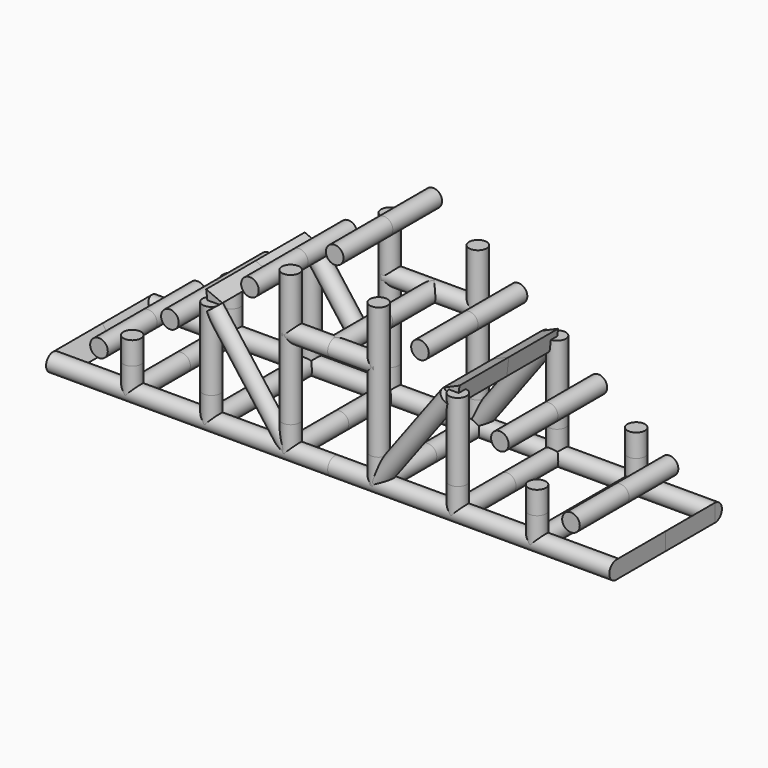
from build123d import *

# Parameters (mm, degrees)
F0_R      = 1.27
F1_DEPTH  = 40.64
F2_DEPTH  = 40.64
F3_R      = 1.27
F4_DEPTH  = 3.81
F6_DEPTH  = 8.89
F7_DEPTH  = 8.89
F11_DEPTH = 8.89
F12_DEPTH = 8.89
F16_DEPTH = 3.302
F17_DEPTH = 11.2522
F18_DEPTH = 19.0246
F5_R      = 1.27
F19_DEPTH = 8.89
F20_DEPTH = 8.89
F21_R     = 1.27
F22_DEPTH = 8.89
F23_DEPTH = 8.89
F24_R     = 1.27
F25_DEPTH = 6.604
F26_DEPTH = 6.604
F27_DEPTH = 8.89
F28_DEPTH = 8.89
F29_R     = 1.2711248992
F30_DEPTH = 17.78
F32_DEPTH = 17.78
F31_R     = 1.27
F33_R     = 1.27
F34_DEPTH = 8.89
F35_DEPTH = 8.89


# Not quite as in the source:
# - the program builds the solid bodies; features that only make, move or delete a surface that nothing else refers to are left out


with BuildPart() as f1:
    # F0 (on Right) → F1 (new body)
    with BuildSketch(Plane.YZ):
        with Locations((-8.89, 0)):
            Circle(F0_R)
    extrude(amount=F1_DEPTH)

    # F5 (on Front) → F11 (join)
    with BuildSketch(Plane.XZ):
        Polygon((40.64, -1.2507883366), (40.64, 1.2892116634), (38.9128, -1.2507883366), align=None)
    extrude(amount=F11_DEPTH)


with BuildPart() as f1b:
    # F0 (on Right) → F1, piece 2 (new body)
    with BuildSketch(Plane.YZ):
        with Locations((8.89, 0)):
            Circle(F0_R)
    extrude(amount=F1_DEPTH)


with BuildPart() as f2:
    # F0 (on Right) → F2 (new body)
    with BuildSketch(Plane.YZ):
        with Locations((-8.89, 0)):
            Circle(F0_R)
    extrude(amount=-F2_DEPTH)

    # F5 (on Front) → F6 (join)
    with BuildSketch(Plane.XZ):
        Polygon((-38.9128, -1.2715099968), (-40.64, 1.2684900032), (-40.64, -1.2715099968), align=None)
    extrude(amount=F6_DEPTH)


with BuildPart() as f2b:
    # F0 (on Right) → F2, piece 2 (new body)
    with BuildSketch(Plane.YZ):
        with Locations((8.89, 0)):
            Circle(F0_R)
    extrude(amount=-F2_DEPTH)


with BuildPart() as f4:
    # F3 (on Top) → F4 (new body)
    with BuildSketch(Plane.XY):
        with Locations((-29.21, -8.8966675103)):
            Circle(F3_R)
    extrude(amount=F4_DEPTH)


with BuildPart() as f4b:
    # F3 (on Top) → F4, piece 2 (new body)
    with BuildSketch(Plane.XY):
        with Locations((-17.78, -8.8966675103)):
            Circle(F3_R)
    extrude(amount=F4_DEPTH)


with BuildPart() as f4c:
    # F3 (on Top) → F4, piece 3 (new body)
    with BuildSketch(Plane.XY):
        with Locations((-6.35, -8.8966675103)):
            Circle(F3_R)
    extrude(amount=F4_DEPTH)


with BuildPart() as f4d:
    # F3 (on Top) → F4, piece 4 (new body)
    with BuildSketch(Plane.XY):
        with Locations((6.35, -8.8966675103)):
            Circle(F3_R)
    extrude(amount=F4_DEPTH)


with BuildPart() as f4e:
    # F3 (on Top) → F4, piece 5 (new body)
    with BuildSketch(Plane.XY):
        with Locations((17.78, -8.8966675103)):
            Circle(F3_R)
    extrude(amount=F4_DEPTH)


with BuildPart() as f4f:
    # F3 (on Top) → F4, piece 6 (new body)
    with BuildSketch(Plane.XY):
        with Locations((29.21, -8.8966675103)):
            Circle(F3_R)
    extrude(amount=F4_DEPTH)


with BuildPart() as f4g:
    # F3 (on Top) → F4, piece 7 (new body)
    with BuildSketch(Plane.XY):
        with Locations((29.21, 8.99035763)):
            Circle(F3_R)
    extrude(amount=F4_DEPTH)


with BuildPart() as f4h:
    # F3 (on Top) → F4, piece 8 (new body)
    with BuildSketch(Plane.XY):
        with Locations((17.78, 8.99035763)):
            Circle(F3_R)
    extrude(amount=F4_DEPTH)


with BuildPart() as f4i:
    # F3 (on Top) → F4, piece 9 (new body)
    with BuildSketch(Plane.XY):
        with Locations((6.35, 8.99035763)):
            Circle(F3_R)
    extrude(amount=F4_DEPTH)


with BuildPart() as f4j:
    # F3 (on Top) → F4, piece 10 (new body)
    with BuildSketch(Plane.XY):
        with Locations((-6.35, 8.99035763)):
            Circle(F3_R)
    extrude(amount=F4_DEPTH)


with BuildPart() as f4k:
    # F3 (on Top) → F4, piece 11 (new body)
    with BuildSketch(Plane.XY):
        with Locations((-17.78, 8.99035763)):
            Circle(F3_R)
    extrude(amount=F4_DEPTH)


with BuildPart() as f4l:
    # F3 (on Top) → F4, piece 12 (new body)
    with BuildSketch(Plane.XY):
        with Locations((-29.21, 8.99035763)):
            Circle(F3_R)
    extrude(amount=F4_DEPTH)


with BuildPart() as f7:
    # F5 (on Front) → F7 (new body)
    with BuildSketch(Plane.XZ):
        Polygon((-38.9128, -1.2715099968), (-40.64, 1.2684900032), (-40.64, -1.2715099968), align=None)
    extrude(amount=-F7_DEPTH)


with BuildPart() as f12:
    # F5 (on Front) → F12 (new body)
    with BuildSketch(Plane.XZ):
        Polygon((40.64, -1.2507883366), (40.64, 1.2892116634), (38.9128, -1.2507883366), align=None)
    extrude(amount=-F12_DEPTH)


with BuildPart() as f16:
    # F16 (new): a face of the model
    f16_faces = [f4.part.faces().sort_by_distance(p)[0] for p in [
        (-29.21, -8.8966675103, 3.81),
    ]]
    extrude(f16_faces, amount=F16_DEPTH)


with BuildPart() as f16b:
    # F16#2 (new): a face of the model
    f16_2_faces = [f4f.part.faces().sort_by_distance(p)[0] for p in [
        (29.21, -8.8966675103, 3.81),
    ]]
    extrude(f16_2_faces, amount=F16_DEPTH)


with BuildPart() as f16c:
    # F16#3 (new): a face of the model
    f16_3_faces = [f4l.part.faces().sort_by_distance(p)[0] for p in [
        (-29.21, 8.99035763, 3.81),
    ]]
    extrude(f16_3_faces, amount=F16_DEPTH)


with BuildPart() as f16d:
    # F16#4 (new): a face of the model
    f16_4_faces = [f4g.part.faces().sort_by_distance(p)[0] for p in [
        (29.21, 8.99035763, 3.81),
    ]]
    extrude(f16_4_faces, amount=F16_DEPTH)


with BuildPart() as f17:
    # F17 (new): a face of the model
    f17_faces = [f4k.part.faces().sort_by_distance(p)[0] for p in [
        (-17.78, 8.99035763, 3.81),
    ]]
    extrude(f17_faces, amount=F17_DEPTH)


with BuildPart() as f17b:
    # F17#2 (new): a face of the model
    f17_2_faces = [f4b.part.faces().sort_by_distance(p)[0] for p in [
        (-17.78, -8.8966675103, 3.81),
    ]]
    extrude(f17_2_faces, amount=F17_DEPTH)


with BuildPart() as f17c:
    # F17#3 (new): a face of the model
    f17_3_faces = [f4h.part.faces().sort_by_distance(p)[0] for p in [
        (17.78, 8.99035763, 3.81),
    ]]
    extrude(f17_3_faces, amount=F17_DEPTH)


with BuildPart() as f17d:
    # F17#4 (new): a face of the model
    f17_4_faces = [f4e.part.faces().sort_by_distance(p)[0] for p in [
        (17.78, -8.8966675103, 3.81),
    ]]
    extrude(f17_4_faces, amount=F17_DEPTH)


with BuildPart() as f18:
    # F18 (new): a face of the model
    f18_faces = [f4c.part.faces().sort_by_distance(p)[0] for p in [
        (-6.35, -8.8966675103, 3.81),
    ]]
    extrude(f18_faces, amount=F18_DEPTH)


with BuildPart() as f18b:
    # F18#2 (new): a face of the model
    f18_2_faces = [f4j.part.faces().sort_by_distance(p)[0] for p in [
        (-6.35, 8.99035763, 3.81),
    ]]
    extrude(f18_2_faces, amount=F18_DEPTH)


with BuildPart() as f18c:
    # F18#3 (new): a face of the model
    f18_3_faces = [f4i.part.faces().sort_by_distance(p)[0] for p in [
        (6.35, 8.99035763, 3.81),
    ]]
    extrude(f18_3_faces, amount=F18_DEPTH)


with BuildPart() as f18d:
    # F18#4 (new): a face of the model
    f18_4_faces = [f4d.part.faces().sort_by_distance(p)[0] for p in [
        (6.35, -8.8966675103, 3.81),
    ]]
    extrude(f18_4_faces, amount=F18_DEPTH)


with BuildPart() as f19:
    # F5 (on Front) → F19 (new body)
    with BuildSketch(Plane.XZ):
        with Locations((-29.21, 0)):
            Circle(F5_R)
    extrude(amount=F19_DEPTH)


with BuildPart() as f19b:
    # F5 (on Front) → F19, piece 2 (new body)
    with BuildSketch(Plane.XZ):
        with Locations((-17.78, 0)):
            Circle(F5_R)
    extrude(amount=F19_DEPTH)


with BuildPart() as f19c:
    # F5 (on Front) → F19, piece 3 (new body)
    with BuildSketch(Plane.XZ):
        with Locations((-6.35, 0)):
            Circle(F5_R)
    extrude(amount=F19_DEPTH)


with BuildPart() as f19d:
    # F5 (on Front) → F19, piece 4 (new body)
    with BuildSketch(Plane.XZ):
        with Locations((6.35, 0)):
            Circle(F5_R)
    extrude(amount=F19_DEPTH)


with BuildPart() as f19e:
    # F5 (on Front) → F19, piece 5 (new body)
    with BuildSketch(Plane.XZ):
        with Locations((17.78, 0)):
            Circle(F5_R)
    extrude(amount=F19_DEPTH)


with BuildPart() as f19f:
    # F5 (on Front) → F19, piece 6 (new body)
    with BuildSketch(Plane.XZ):
        with Locations((29.21, 0)):
            Circle(F5_R)
    extrude(amount=F19_DEPTH)


with BuildPart() as f20:
    # F20 (new): a face of the model
    f20_faces = [f19.part.faces().sort_by_distance(p)[0] for p in [
        (-29.21, 0, 0),
    ]]
    extrude(f20_faces, amount=F20_DEPTH)


with BuildPart() as f20b:
    # F20#2 (new): a face of the model
    f20_2_faces = [f19b.part.faces().sort_by_distance(p)[0] for p in [
        (-17.78, 0, 0),
    ]]
    extrude(f20_2_faces, amount=F20_DEPTH)


with BuildPart() as f20c:
    # F20#3 (new): a face of the model
    f20_3_faces = [f19c.part.faces().sort_by_distance(p)[0] for p in [
        (-6.35, 0, 0),
    ]]
    extrude(f20_3_faces, amount=F20_DEPTH)


with BuildPart() as f20d:
    # F20#4 (new): a face of the model
    f20_4_faces = [f19d.part.faces().sort_by_distance(p)[0] for p in [
        (6.35, 0, 0),
    ]]
    extrude(f20_4_faces, amount=F20_DEPTH)


with BuildPart() as f20e:
    # F20#5 (new): a face of the model
    f20_5_faces = [f19e.part.faces().sort_by_distance(p)[0] for p in [
        (17.78, 0, 0),
    ]]
    extrude(f20_5_faces, amount=F20_DEPTH)


with BuildPart() as f20f:
    # F20#6 (new): a face of the model
    f20_6_faces = [f19f.part.faces().sort_by_distance(p)[0] for p in [
        (29.21, 0, 0),
    ]]
    extrude(f20_6_faces, amount=F20_DEPTH)


with BuildPart() as f22:
    # F21 (on Front) → F22 (new body)
    with BuildSketch(Plane.XZ):
        with Locations((12.3038729653, 18.7193416059)):
            Circle(F21_R)
    extrude(amount=F22_DEPTH)


with BuildPart() as f22b:
    # F21 (on Front) → F22, piece 2 (new body)
    with BuildSketch(Plane.XZ):
        with Locations((0, 26.8041770905)):
            Circle(F21_R)
    extrude(amount=F22_DEPTH)


with BuildPart() as f22c:
    # F21 (on Front) → F22, piece 3 (new body)
    with BuildSketch(Plane.XZ):
        with Locations((-12.2353499755, 18.7193416059)):
            Circle(F21_R)
    extrude(amount=F22_DEPTH)


with BuildPart() as f22d:
    # F21 (on Front) → F22, piece 4 (new body)
    with BuildSketch(Plane.XZ):
        with Locations((-23.786617443, 10.8738057315)):
            Circle(F21_R)
    extrude(amount=F22_DEPTH)


with BuildPart() as f22e:
    # F21 (on Front) → F22, piece 5 (new body)
    with BuildSketch(Plane.XZ):
        with Locations((23.8266456872, 10.8738057315)):
            Circle(F21_R)
    extrude(amount=F22_DEPTH)


with BuildPart() as f22f:
    # F21 (on Front) → F22, piece 6 (new body)
    with BuildSketch(Plane.XZ):
        with Locations((34.0946912766, 3.8956755307)):
            Circle(F21_R)
    extrude(amount=F22_DEPTH)


with BuildPart() as f22g:
    # F21 (on Front) → F22, piece 7 (new body)
    with BuildSketch(Plane.XZ):
        with Locations((-34.0215079486, 3.8956755307)):
            Circle(F21_R)
    extrude(amount=F22_DEPTH)


with BuildPart() as f23:
    # F21 (on Front) → F23 (new body)
    with BuildSketch(Plane.XZ):
        with Locations((0, 26.8041770905)):
            Circle(F21_R)
    extrude(amount=-F23_DEPTH)


with BuildPart() as f23b:
    # F21 (on Front) → F23, piece 2 (new body)
    with BuildSketch(Plane.XZ):
        with Locations((12.3038729653, 18.7193416059)):
            Circle(F21_R)
    extrude(amount=-F23_DEPTH)


with BuildPart() as f23c:
    # F21 (on Front) → F23, piece 3 (new body)
    with BuildSketch(Plane.XZ):
        with Locations((-12.2353499755, 18.7193416059)):
            Circle(F21_R)
    extrude(amount=-F23_DEPTH)


with BuildPart() as f23d:
    # F21 (on Front) → F23, piece 4 (new body)
    with BuildSketch(Plane.XZ):
        with Locations((-23.786617443, 10.8738057315)):
            Circle(F21_R)
    extrude(amount=-F23_DEPTH)


with BuildPart() as f23e:
    # F21 (on Front) → F23, piece 5 (new body)
    with BuildSketch(Plane.XZ):
        with Locations((23.8266456872, 10.8738057315)):
            Circle(F21_R)
    extrude(amount=-F23_DEPTH)


with BuildPart() as f23f:
    # F21 (on Front) → F23, piece 6 (new body)
    with BuildSketch(Plane.XZ):
        with Locations((-34.0215079486, 3.8956755307)):
            Circle(F21_R)
    extrude(amount=-F23_DEPTH)


with BuildPart() as f23g:
    # F21 (on Front) → F23, piece 7 (new body)
    with BuildSketch(Plane.XZ):
        with Locations((34.0946912766, 3.8956755307)):
            Circle(F21_R)
    extrude(amount=-F23_DEPTH)


with BuildPart() as f25:
    # F24 (on Right) → F25 (new body)
    with BuildSketch(Plane.YZ):
        with Locations((8.9446846396, 15.0336446241)):
            Circle(F24_R)
    extrude(amount=F25_DEPTH)


with BuildPart() as f25b:
    # F24 (on Right) → F25, piece 2 (new body)
    with BuildSketch(Plane.YZ):
        with Locations((-8.8928947225, 15.0336446241)):
            Circle(F24_R)
    extrude(amount=F25_DEPTH)


with BuildPart() as f26:
    # F24 (on Right) → F26 (new body)
    with BuildSketch(Plane.YZ):
        with Locations((-8.8928947225, 15.0336446241)):
            Circle(F24_R)
    extrude(amount=-F26_DEPTH)


with BuildPart() as f26b:
    # F24 (on Right) → F26, piece 2 (new body)
    with BuildSketch(Plane.YZ):
        with Locations((8.9446846396, 15.0336446241)):
            Circle(F24_R)
    extrude(amount=-F26_DEPTH)


with BuildPart() as f27:
    # F21 (on Front) → F27 (new body)
    with BuildSketch(Plane.XZ):
        Polygon((18.0123325673, 16.047881465), (15.6810518129, 15.0395511402), (17.7199318668, 13.5247679459), align=None)
    extrude(amount=F27_DEPTH)


with BuildPart() as f27b:
    # F21 (on Front) → F27, piece 2 (new body)
    with BuildSketch(Plane.XZ):
        Polygon((-16.212688792, 15.4057053759), (-18.5507749799, 16.3981533484), (-18.2412170421, 13.8770873272), align=None)
    extrude(amount=F27_DEPTH)


with BuildPart() as f28:
    # F21 (on Front) → F28 (new body)
    with BuildSketch(Plane.XZ):
        Polygon((18.0123325673, 16.047881465), (15.6810518129, 15.0395511402), (17.7199318668, 13.5247679459), align=None)
    extrude(amount=-F28_DEPTH)


with BuildPart() as f28b:
    # F21 (on Front) → F28, piece 2 (new body)
    with BuildSketch(Plane.XZ):
        Polygon((-16.212688792, 15.4057053759), (-18.5507749799, 16.3981533484), (-18.2412170421, 13.8770873272), align=None)
    extrude(amount=-F28_DEPTH)


with BuildPart() as f30:
    # F29 (on face) → F30 (new body)
    with BuildSketch(Plane(origin=(-13.2764674315, 0, 17.6183247795), x_dir=(0.7986331693, 0, 0.6018181294), z_dir=(0.6018181294, 0, -0.7986331693))):
        with Locations((-4.8943031579, -8.8877053931)):
            Circle(F29_R)
    extrude(amount=F30_DEPTH)


with BuildPart() as f30b:
    # F29 (on face) → F30, piece 2 (new body)
    with BuildSketch(Plane(origin=(-13.2764674315, 0, 17.6183247795), x_dir=(0.7986331693, 0, 0.6018181294), z_dir=(0.6018181294, 0, -0.7986331693))):
        with BuildLine():
            ThreePointArc((-3.6765582415, 8.8116565867), (-3.6747477954, 8.8508097002), (-3.6741441224, 8.89))
            ThreePointArc((-3.6741441224, 8.89), (-4.9857485413, 10.1618104461), (-6.2165582415, 8.8116565867))
            Line((-6.2165582415, 8.8116565867), (-6.2165582415, 8.89))
            Line((-6.2165582415, 8.89), (-3.6765582415, 8.89))
            Line((-3.6765582415, 8.89), (-3.6765582415, 8.8116565867))
        make_face()
    extrude(amount=F30_DEPTH)


with BuildPart() as f32:
    # F31 (on face) → F32 (new body)
    with BuildSketch(Plane(origin=(12.7767239819, 0, 17.1973175966), x_dir=(0.8027086827, 0, -0.5963713363), z_dir=(-0.5963713363, 0, -0.8027086827))):
        with BuildLine():
            Line((3.6181592323, 8.89), (6.1581592323, 8.89))
            ThreePointArc((6.1581592323, 8.89), (4.8881592323, 10.16), (3.6181592323, 8.89))
        make_face()
    extrude(amount=F32_DEPTH)


with BuildPart() as f32b:
    # F31 (on face) → F32, piece 2 (new body)
    with BuildSketch(Plane(origin=(12.7767239819, 0, 17.1973175966), x_dir=(0.8027086827, 0, -0.5963713363), z_dir=(-0.5963713363, 0, -0.8027086827))):
        with Locations((4.8881592323, -8.9102927595)):
            Circle(F31_R)
    extrude(amount=F32_DEPTH)


with BuildPart() as f34:
    # F33 (on Front) → F34 (new body)
    with BuildSketch(Plane.XZ):
        with Locations((0, 15.0368586183)):
            Circle(F33_R)
    extrude(amount=F34_DEPTH)


with BuildPart() as f35:
    # F33 (on Front) → F35 (new body)
    with BuildSketch(Plane.XZ):
        with Locations((0, 15.0368586183)):
            Circle(F33_R)
    extrude(amount=-F35_DEPTH)


solid = Compound([f1.part, f1b.part, f2.part, f2b.part, f4.part, f4b.part, f4c.part, f4d.part, f4e.part, f4f.part, f4g.part, f4h.part, f4i.part, f4j.part, f4k.part, f4l.part, f7.part, f12.part, f16.part, f16b.part, f16c.part, f16d.part, f17.part, f17b.part, f17c.part, f17d.part, f18.part, f18b.part, f18c.part, f18d.part, f19.part, f19b.part, f19c.part, f19d.part, f19e.part, f19f.part, f20.part, f20b.part, f20c.part, f20d.part, f20e.part, f20f.part, f22.part, f22b.part, f22c.part, f22d.part, f22e.part, f22f.part, f22g.part, f23.part, f23b.part, f23c.part, f23d.part, f23e.part, f23f.part, f23g.part, f25.part, f25b.part, f26.part, f26b.part, f27.part, f27b.part, f28.part, f28b.part, f30.part, f30b.part, f32.part, f32b.part, f34.part, f35.part])
